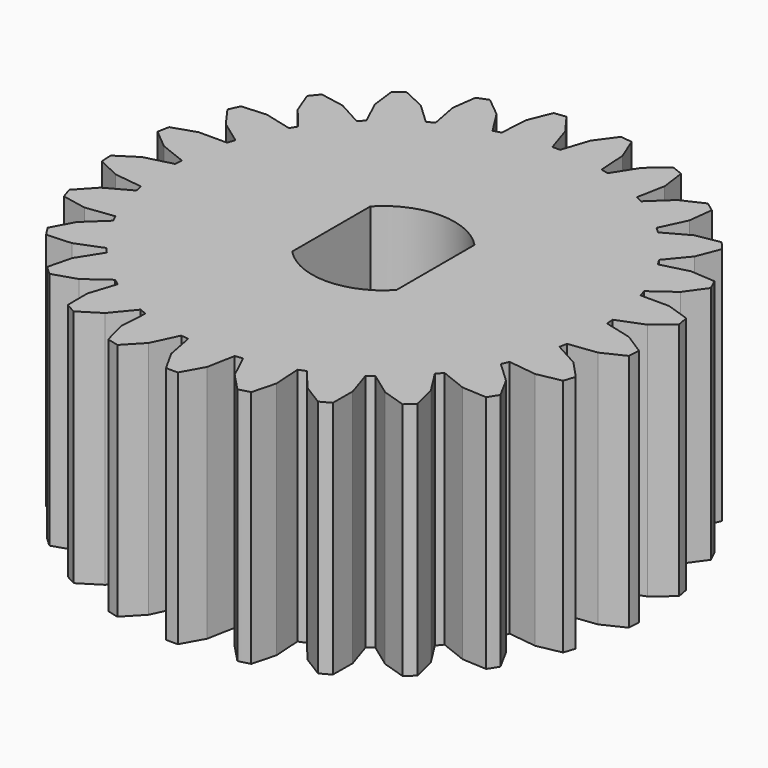
from build123d import *

# Parameters (mm, degrees)
F0_R     = 6.85
F1_DEPTH = 6.2
F3_DEPTH = 25


with BuildPart() as f1:
    # F0 (on Top) → F1 (new body)
    with BuildSketch(Plane.XY):
        Circle(F0_R)
        with BuildLine():
            ThreePointArc((1.35, -1.2649110641), (0, -1.85), (-1.35, -1.2649110641))
            Line((-1.35, -1.2649110641), (-1.35, 1.2649110641))
            ThreePointArc((-1.35, 1.2649110641), (0, 1.85), (1.35, 1.2649110641))
            Line((1.35, 1.2649110641), (1.35, -1.2649110641))
        make_face(mode=Mode.SUBTRACT)
    extrude(amount=F1_DEPTH)

    # F2 (on face) → F3 (cut)
    with BuildSketch(Plane.XY.offset(6.2)):
        with BuildLine():
            Line((0.3280050893, 6.3), (0.7057770525, 6.8135437734))
            ThreePointArc((0.7057770525, 6.8135437734), (0, 6.85), (-0.7057770525, 6.8135437734))
            Line((-0.7057770525, 6.8135437734), (-0.3280050893, 6.3))
            Line((-0.3280050893, 6.3), (-0.1, 5.5982724904))
            ThreePointArc((-0.1, 5.5982724904), (0.0002198008, 5.5998651199), (0.100452053, 5.5996637666))
            Line((0.100452053, 5.5996637666), (0.3280050893, 6.3))
        make_face()
        with BuildLine():
            ThreePointArc((-1.0108556636, 6.7750033821), (-1.7035257271, 6.6347946537), (-2.3780632008, 6.423964151))
            Line((-2.3780632008, 6.423964151), (-1.8844464954, 6.0205023665))
            Line((-1.8844464954, 6.0205023665), (-1.4890920701, 5.3975234769))
            ThreePointArc((-1.4890920701, 5.3975234769), (-1.3924169295, 5.4239897219), (-1.2952835832, 5.4487214421))
            Line((-1.2952835832, 5.4487214421), (-1.2490460829, 6.1836454637))
            Line((-1.2490460829, 6.1836454637), (-1.0108556636, 6.7750033821))
        make_face()
        with BuildLine():
            ThreePointArc((-2.6639726008, 6.3107646115), (-3.3000126676, 6.0027007583), (-3.9009268922, 5.6307432353))
            Line((-3.9009268922, 5.6307432353), (-3.3224811976, 5.3627144274))
            Line((-3.3224811976, 5.3627144274), (-2.7846190089, 4.8576282126))
            ThreePointArc((-2.7846190089, 4.8576282126), (-2.6975629831, 4.9073051017), (-2.6096317882, 4.9554159103))
            Line((-2.6096317882, 4.9554159103), (-2.747615096, 5.6787497411))
            Line((-2.747615096, 5.6787497411), (-2.6639726008, 6.3107646115))
        make_face()
        with BuildLine():
            ThreePointArc((-4.149702342, 5.4499972911), (-4.6891476756, 4.9934350978), (-5.1786810004, 4.4837220137))
            Line((-5.1786810004, 4.4837220137), (-4.5517521871, 4.3679674182))
            Line((-4.5517521871, 4.3679674182), (-3.9051780943, 4.0125103027))
            ThreePointArc((-3.9051780943, 4.0125103027), (-3.8332112335, 4.0822764541), (-3.7600072304, 4.1507433722))
            Line((-3.7600072304, 4.1507433722), (-4.0735413477, 4.8170372873))
            Line((-4.0735413477, 4.8170372873), (-4.149702342, 5.4499972911))
        make_face()
        with BuildLine():
            ThreePointArc((-5.3746910235, 4.2467865972), (-5.7836462897, 3.6704135456), (-6.1310395355, 3.054972048))
            Line((-6.1310395355, 3.054972048), (-5.4950198464, 3.0987649518))
            Line((-5.4950198464, 3.0987649518), (-4.7803604777, 2.9152716134))
            ThreePointArc((-4.7803604777, 2.9152716134), (-4.7280047246, 3.0007433634), (-4.6741275899, 3.0852643626))
            Line((-4.6741275899, 3.0852643626), (-5.143512015, 3.6526526649))
            Line((-5.143512015, 3.6526526649), (-5.3746910235, 4.2467865972))
        make_face()
        with BuildLine():
            ThreePointArc((-6.2619681013, 2.7767346827), (-6.5147371366, 2.1167664115), (-6.6981623082, 1.4342669531))
            Line((-6.6981623082, 1.4342669531), (-6.0930151995, 1.6348556871))
            Line((-6.0930151995, 1.6348556871), (-5.3551752314, 1.6348556871))
            ThreePointArc((-5.3551752314, 1.6348556871), (-5.3257202904, 1.7306625312), (-5.2945553228, 1.8259268463))
            Line((-5.2945553228, 1.8259268463), (-5.8902969058, 2.2587584421))
            Line((-5.8902969058, 2.2587584421), (-6.2619681013, 2.7767346827))
        make_face()
        with BuildLine():
            ThreePointArc((-6.7557826934, 1.1322103161), (-6.8364830897, 0.4301150588), (-6.844414909, -0.2765584093))
            Line((-6.844414909, -0.2765584093), (-6.3081639991, 0.0682224269))
            Line((-6.3081639991, 0.0682224269), (-5.5935046304, 0.2517157653))
            ThreePointArc((-5.5935046304, 0.2517157653), (-5.5888012638, 0.3518378072), (-5.5823066727, 0.451859631))
            Line((-5.5823066727, 0.451859631), (-6.2669727791, 0.7229381192))
            Line((-6.2669727791, 0.7229381192), (-6.7557826934, 1.1322103161))
        make_face()
        with BuildLine():
            ThreePointArc((-6.8251066128, -0.5834549887), (-6.7286676675, -1.2835620049), (-6.560607749, -1.9700065898))
            Line((-6.560607749, -1.9700065898), (-6.1269476548, -1.5026974992))
            Line((-6.1269476548, -1.5026974992), (-5.480373562, -1.1472403837))
            ThreePointArc((-5.480373562, -1.1472403837), (-5.5007172996, -1.0490941802), (-5.5193011641, -0.9505995868))
            Line((-5.5193011641, -0.9505995868), (-6.2498717044, -0.8583070645))
            Line((-6.2498717044, -0.8583070645), (-6.8251066128, -0.5834549887))
        make_face()
        with BuildLine():
            ThreePointArc((-6.4655839828, -2.2624596708), (-6.1980653094, -2.9165881472), (-5.8645734759, -3.539672011))
            Line((-5.8645734759, -3.539672011), (-5.560752656, -2.979197415))
            Line((-5.560752656, -2.979197415), (-5.0228904672, -2.4741112002))
            ThreePointArc((-5.0228904672, -2.4741112002), (-5.0670030372, -2.3841077219), (-5.1094976647, -2.2933291365))
            Line((-5.1094976647, -2.2933291365), (-5.8400682051, -2.3856216588))
            Line((-5.8400682051, -2.3856216588), (-6.4655839828, -2.2624596708))
        make_face()
        with BuildLine():
            ThreePointArc((-5.6998049323, -3.799305691), (-5.278015713, -4.3663543298), (-4.800046483, -4.8869268218))
            Line((-4.800046483, -4.8869268218), (-4.6451551168, -4.2685034004))
            Line((-4.6451551168, -4.2685034004), (-4.2498006916, -3.6455245108))
            ThreePointArc((-4.2498006916, -3.6455245108), (-4.3149103389, -3.5693190073), (-4.3786456357, -3.4919603822))
            Line((-4.3786456357, -3.4919603822), (-5.0633117421, -3.7630388704))
            Line((-5.0633117421, -3.7630388704), (-5.6998049323, -3.799305691))
        make_face()
        with BuildLine():
            ThreePointArc((-4.5758861756, -5.0974273617), (-4.0263289782, -5.5417664115), (-3.4339149162, -5.9271180475))
            Line((-3.4339149162, -5.9271180475), (-3.437685398, -5.2896036187))
            Line((-3.437685398, -5.2896036187), (-3.2096803087, -4.5878761091))
            ThreePointArc((-3.2096803087, -4.5878761091), (-3.2916959548, -4.5302568525), (-3.3726671978, -4.4711789146))
            Line((-3.3726671978, -4.4711789146), (-3.9684087809, -4.9040105104))
            Line((-3.9684087809, -4.9040105104), (-4.5758861756, -5.0974273617))
        make_face()
        with BuildLine():
            ThreePointArc((-3.1644476615, -6.0752589243), (-2.5216531859, -6.3689689283), (-1.8520178461, -6.5948866478))
            Line((-1.8520178461, -6.5948866478), (-2.0142132627, -5.9783385879))
            Line((-2.0142132627, -5.9783385879), (-1.9678839078, -5.2419545785))
            ThreePointArc((-1.9678839078, -5.2419545785), (-2.0616522079, -5.2065419985), (-2.1547716761, -5.169456832))
            Line((-2.1547716761, -5.169456832), (-2.6241561012, -5.7368451343))
            Line((-2.6241561012, -5.7368451343), (-3.1644476615, -6.0752589243))
        make_face()
        with BuildLine():
            ThreePointArc((-1.5541752628, -6.6713596255), (-0.8585326499, -6.795985704), (-0.1537516835, -6.8482742658))
            Line((-0.1537516835, -6.8482742658), (-0.4641807003, -6.2914325567))
            Line((-0.4641807003, -6.2914325567), (-0.6024381235, -5.5666617631))
            ThreePointArc((-0.6024381235, -5.5666617631), (-0.7020672706, -5.5556809624), (-0.8014839253, -5.5429187647))
            Line((-0.8014839253, -5.5429187647), (-1.1150180426, -6.2092126798))
            Line((-1.1150180426, -6.2092126798), (-1.5541752628, -6.6713596255))
        make_face()
        with BuildLine():
            ThreePointArc((0.1537516835, -6.8482742658), (0.8585326499, -6.795985704), (1.5541752628, -6.6713596255))
            Line((1.5541752628, -6.6713596255), (1.1150180426, -6.2092126798))
            Line((1.1150180426, -6.2092126798), (0.8008610637, -5.5415951163))
            ThreePointArc((0.8008610637, -5.5415951163), (0.7016311354, -5.5557360591), (0.6021640081, -5.5680987259))
            Line((0.6021640081, -5.5680987259), (0.4641807003, -6.2914325567))
            Line((0.4641807003, -6.2914325567), (0.1537516835, -6.8482742658))
        make_face()
        with BuildLine():
            ThreePointArc((1.8520178461, -6.5948866478), (2.5216531859, -6.3689689283), (3.1644476615, -6.0752589243))
            Line((3.1644476615, -6.0752589243), (2.6241561012, -5.7368451343))
            Line((2.6241561012, -5.7368451343), (2.1538392049, -5.1683296679))
            ThreePointArc((2.1538392049, -5.1683296679), (2.0612434767, -5.2067038266), (1.9679757624, -5.2434145662))
            Line((1.9679757624, -5.2434145662), (2.0142132627, -5.9783385879))
            Line((2.0142132627, -5.9783385879), (1.8520178461, -6.5948866478))
        make_face()
        with BuildLine():
            ThreePointArc((3.4339149162, -5.9271180475), (4.0263289782, -5.5417664115), (4.5758861756, -5.0974273617))
            Line((4.5758861756, -5.0974273617), (3.9684087809, -4.9040105104))
            Line((3.9684087809, -4.9040105104), (3.3714837076, -4.4703190587))
            ThreePointArc((3.3714837076, -4.4703190587), (3.2913403097, -4.5305152438), (3.2101323618, -4.5892673853))
            Line((3.2101323618, -4.5892673853), (3.437685398, -5.2896036187))
            Line((3.437685398, -5.2896036187), (3.4339149162, -5.9271180475))
        make_face()
        with BuildLine():
            ThreePointArc((4.800046483, -4.8869268218), (5.278015713, -4.3663543298), (5.6998049323, -3.799305691))
            Line((5.6998049323, -3.799305691), (5.0633117421, -3.7630388704))
            Line((5.0633117421, -3.7630388704), (4.3772854895, -3.4914218623))
            ThreePointArc((4.3772854895, -3.4914218623), (4.3146301263, -3.5696577262), (4.2505845388, -3.6467596565))
            Line((4.2505845388, -3.6467596565), (4.6451551168, -4.2685034004))
            Line((4.6451551168, -4.2685034004), (4.800046483, -4.8869268218))
        make_face()
        with BuildLine():
            ThreePointArc((5.8645734759, -3.539672011), (6.1980653094, -2.9165881472), (6.4655839828, -2.2624596708))
            Line((6.4655839828, -2.2624596708), (5.8400682051, -2.3856216588))
            Line((5.8400682051, -2.3856216588), (5.1080463256, -2.2931457897))
            ThreePointArc((5.1080463256, -2.2931457897), (5.066815864, -2.3845054853), (5.0239568568, -2.4751126066))
            Line((5.0239568568, -2.4751126066), (5.560752656, -2.979197415))
            Line((5.560752656, -2.979197415), (5.8645734759, -3.539672011))
        make_face()
        with BuildLine():
            ThreePointArc((6.560607749, -1.9700065898), (6.7286676675, -1.2835620049), (6.8251066128, -0.5834549887))
            Line((6.8251066128, -0.5834549887), (6.2498717044, -0.8583070645))
            Line((6.2498717044, -0.8583070645), (5.5178498249, -0.9507829336))
            ThreePointArc((5.5178498249, -0.9507829336), (5.5006349265, -1.0495259952), (5.4816554886, -1.1479451288))
            Line((5.4816554886, -1.1479451288), (6.1269476548, -1.5026974992))
            Line((6.1269476548, -1.5026974992), (6.560607749, -1.9700065898))
        make_face()
        with BuildLine():
            ThreePointArc((6.844414909, -0.2765584093), (6.8364830897, 0.4301150588), (6.7557826934, 1.1322103161))
            Line((6.7557826934, 1.1322103161), (6.2669727791, 0.7229381192))
            Line((6.2669727791, 0.7229381192), (5.5809465265, 0.451321111))
            ThreePointArc((5.5809465265, 0.451321111), (5.5888288666, 0.3513990731), (5.5949215459, 0.2513519632))
            Line((5.5949215459, 0.2513519632), (6.3081639991, 0.0682224269))
            Line((6.3081639991, 0.0682224269), (6.844414909, -0.2765584093))
        make_face()
        with BuildLine():
            ThreePointArc((6.6981623082, 1.4342669531), (6.5147371366, 2.1167664115), (6.2619681013, 2.7767346827))
            Line((6.2619681013, 2.7767346827), (5.8902969058, 2.2587584421))
            Line((5.8902969058, 2.2587584421), (5.2933718326, 1.8250669903))
            ThreePointArc((5.2933718326, 1.8250669903), (5.3258561348, 1.7302444453), (5.3566381058, 1.6348556871))
            Line((5.3566381058, 1.6348556871), (6.0930151995, 1.6348556871))
            Line((6.0930151995, 1.6348556871), (6.6981623082, 1.4342669531))
        make_face()
        with BuildLine():
            ThreePointArc((6.1310395355, 3.054972048), (5.7836462897, 3.6704135456), (5.3746910235, 4.2467865972))
            Line((5.3746910235, 4.2467865972), (5.143512015, 3.6526526649))
            Line((5.143512015, 3.6526526649), (4.6731951187, 3.0841371985))
            ThreePointArc((4.6731951187, 3.0841371985), (4.7282402749, 3.0003721955), (4.7817773932, 2.9156354155))
            Line((4.7817773932, 2.9156354155), (5.4950198464, 3.0987649518))
            Line((5.4950198464, 3.0987649518), (6.1310395355, 3.054972048))
        make_face()
        with BuildLine():
            ThreePointArc((5.1786810004, 4.4837220137), (4.6891476756, 4.9934350978), (4.149702342, 5.4499972911))
            Line((4.149702342, 5.4499972911), (4.0735413477, 4.8170372873))
            Line((4.0735413477, 4.8170372873), (3.7593843688, 4.1494197239))
            ThreePointArc((3.7593843688, 4.1494197239), (3.8335316893, 4.0819755262), (3.9064600208, 4.0132150478))
            Line((3.9064600208, 4.0132150478), (4.5517521871, 4.3679674182))
            Line((4.5517521871, 4.3679674182), (5.1786810004, 4.4837220137))
        make_face()
        with BuildLine():
            ThreePointArc((3.9009268922, 5.6307432353), (3.3000126676, 6.0027007583), (2.6639726008, 6.3107646115))
            Line((2.6639726008, 6.3107646115), (2.747615096, 5.6787497411))
            Line((2.747615096, 5.6787497411), (2.6093576729, 4.9539789475))
            ThreePointArc((2.6093576729, 4.9539789475), (2.6979482089, 4.907093322), (2.7856853984, 4.8586296191))
            Line((2.7856853984, 4.8586296191), (3.3224811976, 5.3627144274))
            Line((3.3224811976, 5.3627144274), (3.9009268922, 5.6307432353))
        make_face()
        with BuildLine():
            ThreePointArc((2.3780632008, 6.423964151), (1.7035257271, 6.6347946537), (1.0108556636, 6.7750033821))
            Line((1.0108556636, 6.7750033821), (1.2490460829, 6.1836454637))
            Line((1.2490460829, 6.1836454637), (1.2953754378, 5.4472614543))
            ThreePointArc((1.2953754378, 5.4472614543), (1.3928427201, 5.4238803974), (1.4898759174, 5.3987586226))
            Line((1.4898759174, 5.3987586226), (1.8844464954, 6.0205023665))
            Line((1.8844464954, 6.0205023665), (2.3780632008, 6.423964151))
        make_face()
    extrude(amount=-F3_DEPTH, mode=Mode.SUBTRACT)


solid = f1.part
